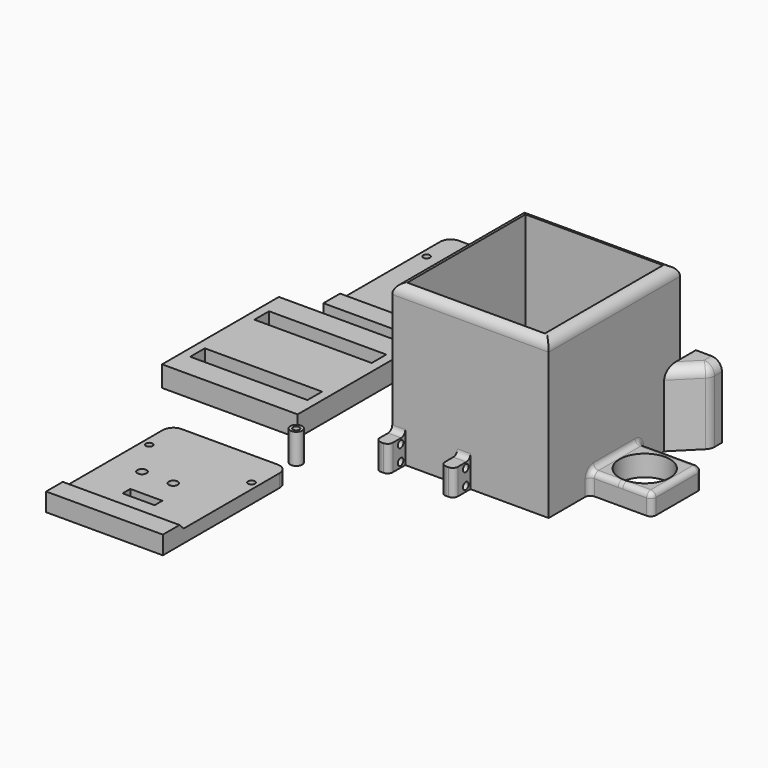
from build123d import *

# Parameters (mm, degrees)
F0_W         = 76.2
F0_H         = 76.2
F1_DEPTH     = 3.81
F2_W         = 6.35
F2_H         = 12.7
F3_DEPTH     = 10.16
F4_R         = 1.7145
F5_DEPTH     = 50.8
F6_ANGLE     = 90
F7_W         = 4.445
F7_H         = 76.2
F8_DEPTH     = 76.2
F9_W         = 4.445
F9_H         = 76.2
F10_DEPTH    = 71.755
F11_W        = 4.7111754219
F11_H        = 76.2
F12_DEPTH    = 73.533
F14_T1_DEPTH = 105.41
F14_T3_DEPTH = 101.6
F15_W        = 12.7
F15_H        = 35.56
F16_DEPTH    = 9.652
F17_SIZE     = 12.69999
F18_R        = 5.08
F19_W        = 30.48
F19_H        = 10.16
F20_DEPTH    = 30.48
F21_R        = 12.2555
F22_DEPTH    = 25.4
F23_F1_R     = 2.54
F23_F2_R     = 2.54
F24_R        = 2.54
F25_W        = 66.04
F25_H        = 71.12
F26_DEPTH    = 10.16
F27_W        = 57.15
F27_H        = 8.89
F28_DEPTH    = 6.35
F29_R        = 2.921
F30_DEPTH    = 14.605
F31_R        = 1.5875
F32_DEPTH    = 25.4
F33_W        = 56.896
F33_H        = 76.2
F34_DEPTH    = 6.35
F35_R        = 5.08
F36_W        = 56.896
F36_H        = 12.7
F37_DEPTH    = 2.54
F38_SIZE     = 2.53999
F39_R        = 1.651
F39_R_2      = 2.2225
F40_DEPTH    = 25.4
F42_W        = 15.621
F42_H        = 4.699
F43_DEPTH    = 25.4


# Not quite as in the source:
# - a fillet or chamfer that OpenCascade refuses, or shapes differently, is made with other operations: its cross-section is extruded or revolved along the edge and cut away or added
# - a fillet or chamfer is up to 0.001 mm smaller than in the source, because OpenCascade refuses the exact size


with BuildPart() as f1:
    # F0 (on Top) → F1 (new body)
    with BuildSketch(Plane.XY):
        with Locations((-2.667912658, -5.7110823691)):
            Rectangle(F0_W, F0_H)
    extrude(amount=F1_DEPTH)

    # F2 (on face) → F3 (join)
    with BuildSketch(Plane.XY.offset(3.81)):
        with Locations((-37.592912658, -37.4610823691)):
            Rectangle(F2_W, F2_H)
        with Locations((-5.842912658, -37.4610823691)):
            Rectangle(F2_W, F2_H)
    extrude(amount=F3_DEPTH)

    # F4 (on face) → F5 (cut)
    with BuildSketch(Plane.YZ.offset(-2.667912658)):
        with Locations((-41.2710823691, 6.6548)):
            Circle(F4_R)
        with Locations((-33.6510823691, 6.6548)):
            Circle(F4_R)
    extrude(amount=-F5_DEPTH, mode=Mode.SUBTRACT)


with BuildPart() as f1_1:
    # F6: moved
    add(f1.part.rotate(Axis((-2.667912658, -43.8110823691, 0), (1, 0, 0)), F6_ANGLE))

    # F7 (on face) → F8 (join)
    with BuildSketch(Plane(origin=(0, -43.8110823691, 0), x_dir=(-1, 0, 0), z_dir=(0, 1, 0))):
        with Locations((38.545412658, 38.1)):
            Rectangle(F7_W, F7_H)
    extrude(amount=F8_DEPTH)

    # F9 (on face) → F10 (join)
    with BuildSketch(Plane.YZ.offset(-36.322912658)):
        with Locations((30.1664176309, 38.1)):
            Rectangle(F9_W, F9_H)
    extrude(amount=F10_DEPTH)

    # F11 (on face) → F12 (join)
    with BuildSketch(Plane.XZ.offset(-27.9439176309)):
        with Locations((33.076499631, 38.1)):
            Rectangle(F11_W, F11_H)
    extrude(amount=F12_DEPTH)

    # F14: fillet of radius 5.08 on 4 edges, made by hand

    # F14_s2 → F14_t1 (cut)
    with BuildSketch(Plane.XZ.offset(-45.0889176309)):
        with BuildLine():
            ThreePointArc((-35.687912658, 76.2), (-39.2800151065, 74.7121024484), (-40.767912658, 71.12))
            Line((-40.767912658, 71.12), (-40.767912658, 76.2))
            Line((-40.767912658, 76.2), (-35.687912658, 76.2))
        make_face()
        with BuildLine():
            ThreePointArc((30.352087342, 76.2), (33.9441897904, 74.7121024484), (35.432087342, 71.12))
            Line((35.432087342, 71.12), (35.432087342, 76.2))
            Line((35.432087342, 76.2), (30.352087342, 76.2))
        make_face()
    extrude(amount=F14_T1_DEPTH, mode=Mode.SUBTRACT)

    # F14_s4 → F14_t3 (cut)
    with BuildSketch(Plane.YZ.offset(-53.467912658)):
        with BuildLine():
            ThreePointArc((-42.5410823691, 76.2), (-46.1331848175, 74.7121024484), (-47.6210823691, 71.12))
            Line((-47.6210823691, 71.12), (-47.6210823691, 76.2))
            Line((-47.6210823691, 76.2), (-42.5410823691, 76.2))
        make_face()
        with BuildLine():
            ThreePointArc((27.3089176309, 76.2), (30.9010200793, 74.7121024484), (32.3889176309, 71.12))
            Line((32.3889176309, 71.12), (32.3889176309, 76.2))
            Line((32.3889176309, 76.2), (27.3089176309, 76.2))
        make_face()
    extrude(amount=F14_T3_DEPTH, mode=Mode.SUBTRACT)

    # F15 (on face) → F16 (join, symmetric)
    with BuildSketch(Plane(origin=(0, 32.3889176309, 0), x_dir=(-1, 0, 0), z_dir=(0, 1, 0))):
        with Locations((-41.782087342, 17.78)):
            Rectangle(F15_W, F15_H)
        with Locations((47.117912658, 17.78)):
            Rectangle(F15_W, F15_H)
    extrude(amount=F16_DEPTH, both=True)

    # F17 (size 12.7 in the source; OpenCascade refuses exactly that, so slightly less here)
    f17_edges = [f1_1.edges().sort_by_distance(p)[0] for p in [
        (48.132087, 22.736918, 17.78),
        (-53.467913, 22.736918, 17.78),
    ]]
    chamfer(f17_edges, length=F17_SIZE)

    # F18
    f18_edges = [f1_1.edges().sort_by_distance(p)[0] for p in [
        (-53.467913, 38.738913, 35.56),
        (48.132087, 38.738913, 35.56),
        (-47.117918, 29.086913, 35.56),
        (-53.467913, 35.436908, 17.78),
        (41.782092, 29.086913, 35.56),
        (48.132087, 35.436908, 17.78),
    ]]
    fillet(f18_edges, radius=F18_R)

    # F19 (on face) → F20 (join)
    with BuildSketch(Plane.YZ.offset(35.432087342)):
        with Locations((-7.6160823691, 5.08)):
            Rectangle(F19_W, F19_H)
    extrude(amount=F20_DEPTH)

    # F21 (on face) → F22 (cut)
    with BuildSketch(Plane.XY.offset(10.16)):
        with Locations((50.672087342, -8.1120058894)):
            Circle(F21_R)
    extrude(amount=-F22_DEPTH, mode=Mode.SUBTRACT)

    # F23: fillet of radius 2.54 on 6 edges, made by hand

    # F23_f1
    f23_f1_edges = [f1_1.edges().sort_by_distance(p)[0] for p in [
        (50.672087342, -22.8560823691, 10.16),
        (65.912087342, -7.6160823691, 10.16),
        (50.672087342, 7.6239176309, 10.16),
        (65.912087342, -22.8560823691, 5.08),
        (65.912087342, 7.6239176309, 5.08),
    ]]
    fillet(f23_f1_edges, radius=F23_F1_R)

    # F23_f2
    f23_f2_edges = [f1_1.edges().sort_by_distance(p)[0] for p in [
        (35.432087342, -22.8560823691, 3.81),
        (35.432087342, -22.1121335933, 9.4160512242),
    ]]
    fillet(f23_f2_edges, radius=F23_F2_R)

    # F24
    f24_edges = [f1_1.edges().sort_by_distance(p)[0] for p in [
        (-5.842913, -47.621082, 12.7),
        (-37.592913, -47.621082, 12.7),
        (-34.417913, -57.781082, 6.35),
        (-40.767913, -57.781082, 6.35),
        (-9.017913, -57.781082, 6.35),
        (-2.667913, -57.781082, 6.35),
    ]]
    fillet(f24_edges, radius=F24_R)


with BuildPart() as f26:
    # F25 (on Top) → F26 (new body)
    with BuildSketch(Plane.XY):
        with Locations((-113.3317090571, -20.2597667474)):
            Rectangle(F25_W, F25_H)
    extrude(amount=F26_DEPTH)

    # F27 (on face) → F28 (cut)
    with BuildSketch(Plane.XY.offset(10.16)):
        with Locations((-113.3317090571, -0.7017667474)):
            Rectangle(F27_W, F27_H)
        with Locations((-113.3317090571, -39.8177667474)):
            Rectangle(F27_W, F27_H)
    extrude(amount=-F28_DEPTH, mode=Mode.SUBTRACT)


with BuildPart() as f30:
    # F29 (on Top) → F30 (new body)
    with BuildSketch(Plane.XY):
        with Locations((-68.1654065847, -71.8291476369)):
            Circle(F29_R)
    extrude(amount=F30_DEPTH)

    # F31 (on face) → F32 (cut)
    with BuildSketch(Plane.XY.offset(14.605)):
        with Locations((-68.1654065847, -71.8291476369)):
            Circle(F31_R)
    extrude(amount=-F32_DEPTH, mode=Mode.SUBTRACT)


with BuildPart() as f34:
    # F33 (on Top) → F34 (new body)
    with BuildSketch(Plane.XY):
        with Locations((-102.9605381191, 61.8491081373)):
            Rectangle(F33_W, F33_H)
    extrude(amount=F34_DEPTH)

    # F35
    f35_edges = [f34.edges().sort_by_distance(p)[0] for p in [
        (-131.408538, 99.949108, 3.175),
        (-74.512538, 99.949108, 3.175),
    ]]
    fillet(f35_edges, radius=F35_R)

    # F36 (on face) → F37 (join)
    with BuildSketch(Plane.XY.offset(6.35)):
        with Locations((-102.9605381191, 30.0991081373)):
            Rectangle(F36_W, F36_H)
    extrude(amount=F37_DEPTH)

    # F38 (size 2.54 in the source; OpenCascade refuses exactly that, so slightly less here)
    f38_edges = [f34.edges().sort_by_distance(p)[0] for p in [
        (-102.960538, 36.449108, 8.89),
    ]]
    chamfer(f38_edges, length=F38_SIZE)

    # F39 (on face) → F40 (cut)
    with BuildSketch(Plane.XY.offset(6.35)):
        with Locations((-78.0685381191, 82.1691081373)):
            Circle(F39_R)
        with Locations((-127.8525381191, 82.1691081373)):
            Circle(F39_R)
        with Locations((-100.9285381191, 63.1191081373)):
            Circle(F39_R_2)
        with Locations((-116.1685381191, 63.1191081373)):
            Circle(F39_R_2)
    extrude(amount=-F40_DEPTH, mode=Mode.SUBTRACT)


with BuildPart() as f41_1:
    # F41: copy of F34
    add(f34.part.moved(Location((-135.128, 0, -124.714))))

    # F42 (on face) → F43 (cut)
    with BuildSketch(Plane.XY.offset(-118.364)):
        with Locations((-238.0885381191, 46.8827777416)):
            Rectangle(F42_W, F42_H)
    extrude(amount=-F43_DEPTH, mode=Mode.SUBTRACT)


solid = Compound([f1_1.part, f26.part, f30.part, f34.part, f41_1.part])
